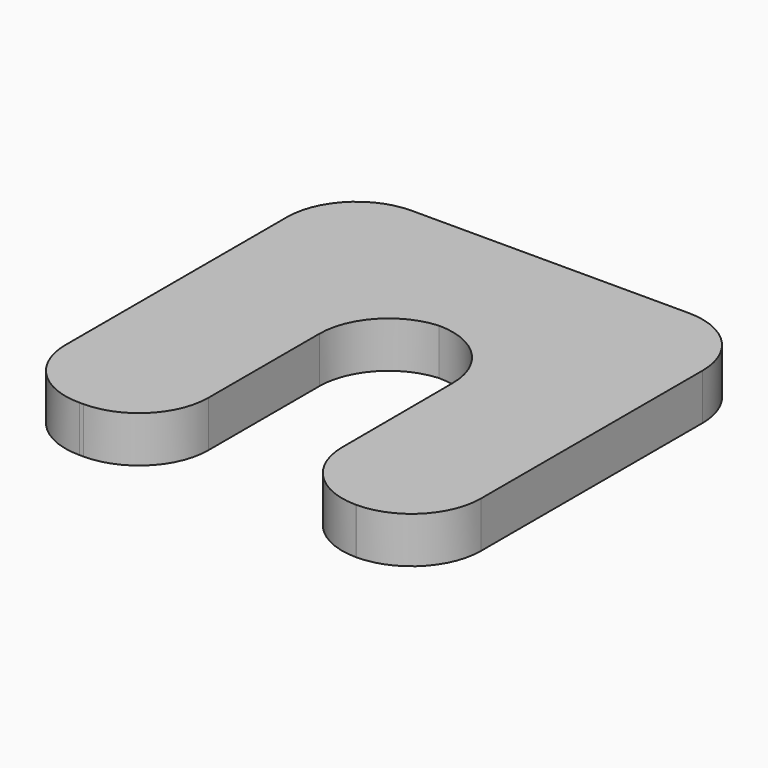
from build123d import *

# Parameters (mm, degrees)
F1_DEPTH    = 10
F2_R        = 15
F3_R        = 15
F4_R        = 15
F5_R        = 15
F6_T1_DEPTH = 10


# Not quite as in the source:
# - a fillet or chamfer that OpenCascade refuses, or shapes differently, is made with other operations: its cross-section is extruded or revolved along the edge and cut away or added


with BuildPart() as f1:
    # F0 (on Top) → F1 (new body)
    with BuildSketch(Plane.XY):
        Polygon((0, 90), (0, 0), (30.9630036354, 0), (30.9630036354, 60), (59.8146165162, 60), (60, 0), (90, 0), (90, 90), align=None)
    extrude(amount=F1_DEPTH)

    # F2
    f2_edges = [f1.edges().sort_by_distance(p)[0] for p in [
        (0, 90, 5),
        (90, 90, 5),
    ]]
    fillet(f2_edges, radius=F2_R)

    # F3
    f3_edges = [f1.edges().sort_by_distance(p)[0] for p in [
        (0, 0, 5),
        (30.963004, 0, 5),
    ]]
    fillet(f3_edges, radius=F3_R)

    # F4
    f4_edges = [f1.edges().sort_by_distance(p)[0] for p in [
        (60, 0, 5),
        (90, 0, 5),
    ]]
    fillet(f4_edges, radius=F4_R)

    # F5
    f5_edges = [f1.edges().sort_by_distance(p)[0] for p in [
        (59.814617, 60, 5),
    ]]
    fillet(f5_edges, radius=F5_R)

    # F6: fillet of radius 15 on 1 edges, made by hand

    # F6_s2 → F6_t1 (join)
    with BuildSketch(Plane.XY):
        with BuildLine():
            ThreePointArc((44.8608907894, 60), (34.9736521375, 55.2500561159), (30.9630036354, 45.0405432159))
            Line((30.9630036354, 45.0405432159), (30.9630036354, 60))
            Line((30.9630036354, 60), (44.8608907894, 60))
        make_face()
    extrude(amount=F6_T1_DEPTH)


solid = f1.part
